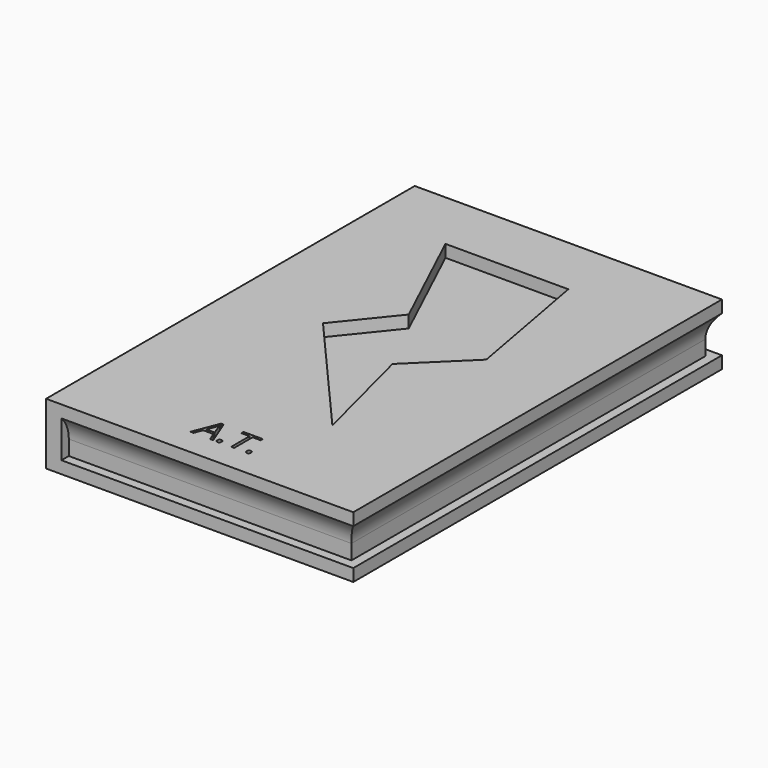
from build123d import *

# Parameters (mm, degrees)
F0_W          = 50
F0_H          = 75
F1_DEPTH      = 10
F2_W          = 47.5
F2_H          = 6
F5_DEPTH      = 1.5
F4_W          = 75
F4_H          = 6
F6_DEPTH      = 1.5
F3_W          = 47.5
F3_H          = 6
F7_DEPTH      = 1.5
F8_TEXT_SIZE  = 5.8516960775
F9_DEPTH      = 2
F10_T1_DEPTH  = 46
F10_T3_DEPTH  = 72
F10_T9_DEPTH  = 80.9267855357
F10_T14_DEPTH = 54.9267855357
F10_T22_DEPTH = 54.9267855357
F10_T27_DEPTH = 80.9267855357


# Not quite as in the source:
# - a fillet or chamfer that OpenCascade refuses, or shapes differently, is made with other operations: its cross-section is extruded or revolved along the edge and cut away or added
# - Text() gives the source's letters only with a copy of the font that has no kerning and outlines rounded to 1/6400 em; it was checked with that copy


with BuildPart() as f1:
    # F0 (on Top) → F1 (new body)
    with BuildSketch(Plane.XY):
        with Locations((-36.4217554219, -16.0150824268)):
            Rectangle(F0_W, F0_H)
    extrude(amount=F1_DEPTH)

    # F2 (on face) → F5 (cut)
    with BuildSketch(Plane.XZ.offset(53.5150824268)):
        with Locations((-35.1717554219, 5)):
            Rectangle(F2_W, F2_H)
    extrude(amount=-F5_DEPTH, mode=Mode.SUBTRACT)

    # F4 (on face) → F6 (cut)
    with BuildSketch(Plane.YZ.offset(-11.4217554219)):
        with Locations((-16.0150824268, 5)):
            Rectangle(F4_W, F4_H)
    extrude(amount=-F6_DEPTH, mode=Mode.SUBTRACT)

    # F3 (on face) → F7 (cut)
    with BuildSketch(Plane(origin=(0, 21.4849175732, 0), x_dir=(-1, 0, 0), z_dir=(0, 1, 0))):
        with Locations((35.1717554219, 5)):
            Rectangle(F3_W, F3_H)
    extrude(amount=-F7_DEPTH, mode=Mode.SUBTRACT)

    # F8 (on face) → F9 (cut)
    with BuildSketch(Plane.XY.offset(10)):
        Polygon((-28.4217554219, 11.4849175732), (-48.4217554219, 11.4849175732), (-39.9146528316, -6.6156129582), (-46.9243637234, -15.3012097358), (-28.4217554219, -36.5150824268), (-33.0267832468, -18.5346256266), (-24.4598607939, -10.1554010695), align=None)
        with Locations((-41.4217554219, -49.1486693687)):
            Text('A.T.', F8_TEXT_SIZE, font='Open Sans', text_align=(TextAlign.LEFT, TextAlign.BOTTOM))
    extrude(amount=-F9_DEPTH, mode=Mode.SUBTRACT)

    # F10: fillet of radius 5 on 3 edges, made by hand

    # F10_s2 → F10_t1 (join)
    with BuildSketch(Plane.YZ.offset(-58.9217554219)):
        with BuildLine():
            ThreePointArc((-53.5150824268, 8), (-52.4053101982, 6.3657774588), (-52.0150824268, 4.4292857857))
            Line((-52.0150824268, 4.4292857857), (-52.0150824268, 8))
            Line((-52.0150824268, 8), (-53.5150824268, 8))
        make_face()
        with BuildLine():
            ThreePointArc((21.4849175732, 8), (20.3751453445, 6.3657774588), (19.9849175732, 4.4292857857))
            Line((19.9849175732, 4.4292857857), (19.9849175732, 8))
            Line((19.9849175732, 8), (21.4849175732, 8))
        make_face()
    extrude(amount=F10_T1_DEPTH)

    # F10_s4 → F10_t3 (join)
    with BuildSketch(Plane.XZ.offset(-19.9849175732)):
        with BuildLine():
            ThreePointArc((-11.4217554219, 8), (-12.5315276506, 6.3657774588), (-12.9217554219, 4.4292857857))
            Line((-12.9217554219, 4.4292857857), (-12.9217554219, 8))
            Line((-12.9217554219, 8), (-11.4217554219, 8))
        make_face()
    extrude(amount=F10_T3_DEPTH)


with BuildPart() as f10_tool7:
    # F10_s8 → F10_t9 (new body)
    with BuildSketch(Plane.XZ.offset(-19.9849175732)):
        with BuildLine():
            ThreePointArc((-11.4217554219, 8), (-12.5315276506, 6.3657774588), (-12.9217554219, 4.4292857857))
            Line((-12.9217554219, 4.4292857857), (-12.9217554219, 8))
            Line((-12.9217554219, 8), (-11.4217554219, 8))
        make_face()
    extrude(amount=F10_T9_DEPTH)

    split(bisect_by=Plane.XZ.offset(53.5150824268), keep=Keep.BOTTOM)

    split(bisect_by=Plane.XZ.offset(52.0150824268), keep=Keep.TOP)


with BuildPart() as f10_tool12:
    # F10_s13 → F10_t14 (new body)
    with BuildSketch(Plane.YZ.offset(-3.9949698862)):
        with BuildLine():
            ThreePointArc((-53.5150824268, 8), (-52.4053101982, 6.3657774588), (-52.0150824268, 4.4292857857))
            Line((-52.0150824268, 4.4292857857), (-52.0150824268, 8))
            Line((-52.0150824268, 8), (-53.5150824268, 8))
        make_face()
    extrude(amount=-F10_T14_DEPTH)

    split(bisect_by=Plane.YZ.offset(-11.4217554219), keep=Keep.BOTTOM)

    split(bisect_by=Plane.YZ.offset(-12.9217554219), keep=Keep.TOP)


with BuildPart() as f10_tool7_1:
    add(f10_tool7.part)

    # F10_t17: intersect F10_tool12
    add(f10_tool12.part, mode=Mode.INTERSECT)


with BuildPart() as f1_1:
    add(f1.part)

    # F10_t5: union F10_tool7
    add(f10_tool7_1.part)


with BuildPart() as f10_tool20:
    # F10_s21 → F10_t22 (new body)
    with BuildSketch(Plane.YZ.offset(-58.9217554219)):
        with BuildLine():
            ThreePointArc((21.4849175732, 8), (20.3751453445, 6.3657774588), (19.9849175732, 4.4292857857))
            Line((19.9849175732, 4.4292857857), (19.9849175732, 8))
            Line((19.9849175732, 8), (21.4849175732, 8))
        make_face()
    extrude(amount=F10_T22_DEPTH)

    split(bisect_by=Plane.YZ.offset(-11.4217554219), keep=Keep.BOTTOM)

    split(bisect_by=Plane.YZ.offset(-12.9217554219), keep=Keep.TOP)


with BuildPart() as f10_tool25:
    # F10_s26 → F10_t27 (new body)
    with BuildSketch(Plane.XZ.offset(-28.9117031088)):
        with BuildLine():
            ThreePointArc((-11.4217554219, 8), (-12.5315276506, 6.3657774588), (-12.9217554219, 4.4292857857))
            Line((-12.9217554219, 4.4292857857), (-12.9217554219, 8))
            Line((-12.9217554219, 8), (-11.4217554219, 8))
        make_face()
    extrude(amount=F10_T27_DEPTH)

    split(bisect_by=Plane.XZ.offset(-21.4849175732), keep=Keep.TOP)

    split(bisect_by=Plane.XZ.offset(-19.9849175732), keep=Keep.BOTTOM)


with BuildPart() as f10_tool20_1:
    add(f10_tool20.part)

    # F10_t30: intersect F10_tool25
    add(f10_tool25.part, mode=Mode.INTERSECT)


with BuildPart() as f1_2:
    add(f1_1.part)

    # F10_t18: union F10_tool20
    add(f10_tool20_1.part)


solid = f1_2.part
